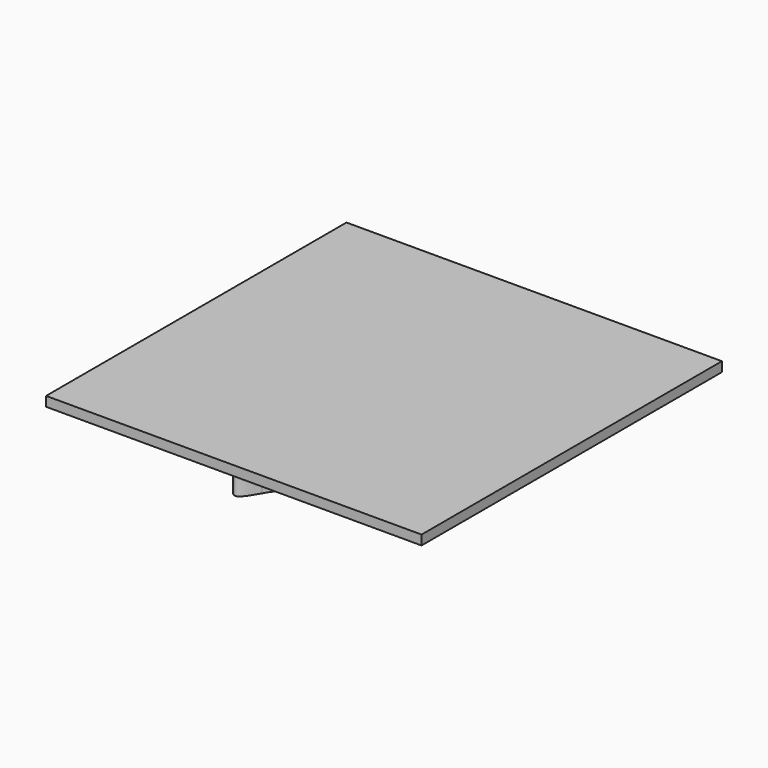
from build123d import *

# Parameters (mm, degrees)
F1_DEPTH = 25.4
F2_W     = 495.3
F2_H     = 495.3
F3_DEPTH = 12.7


# Not quite as in the source:
# - ends of sketch curves that miss each other by under 0.0002 mm in the source are joined


with BuildPart() as f1:
    # F0 (on Top) → F1 (new body)
    with BuildSketch(Plane.XY):
        with BuildLine():
            add(Edge.make_bspline(
                [(-4.6872398, -132.8896504), (2.565146, -134.5904598), (20.1811382, -134.4409808), (32.0904362, -132.5775352)],
                knots=[0, 0, 0, 0, 1, 1, 1, 1], degree=3))
            add(Edge.make_bspline(
                [(32.0904362, -132.5775352), (45.5382884, -130.47345), (63.2073666, -117.8832542), (63.2073666, -110.4049862)],
                knots=[0, 0, 0, 0, 1, 1, 1, 1], degree=3))
            add(Edge.make_bspline(
                [(63.2073666, -110.4049862), (63.2073666, -108.6564248), (65.2077436, -106.314367), (67.652646, -105.2003992)],
                knots=[0, 0, 0, 0, 1, 1, 1, 1], degree=3))
            add(Edge.make_bspline(
                [(67.652646, -105.2003992), (71.0041252, -103.6733512), (72.0979254, -101.8173224), (72.0979254, -97.657285)],
                knots=[0, 0, 0, 0, 1, 1, 1, 1], degree=3))
            add(Edge.make_bspline(
                [(72.0979254, -97.657285), (72.0979254, -93.98508), (74.1760264, -89.6034784), (78.3109432, -84.557362)],
                knots=[0, 0, 0, 0, 1, 1, 1, 1], degree=3))
            add(Edge.make_bspline(
                [(78.3109432, -84.557362), (81.7281068, -80.3871392), (85.0385396, -74.2513628), (85.667469, -70.922261)],
                knots=[0, 0, 0, 0, 1, 1, 1, 1], degree=3))
            add(Edge.make_bspline(
                [(85.667469, -70.922261), (86.2963476, -67.5931846), (88.1013732, -63.3937772), (89.6785608, -61.5902756)],
                knots=[0, 0, 0, 0, 1, 1, 1, 1], degree=3))
            add(Edge.make_bspline(
                [(89.6785608, -61.5902756), (96.3774298, -53.9301944), (96.9903826, -27.6993604), (90.744548, -15.9731456)],
                knots=[0, 0, 0, 0, 1, 1, 1, 1], degree=3))
            add(Edge.make_bspline(
                [(90.744548, -15.9731456), (89.441782, -13.5272526), (86.5961184, -7.5253342), (84.4208624, -2.6355294)],
                knots=[0, 0, 0, 0, 1, 1, 1, 1], degree=3))
            add(Edge.make_bspline(
                [(84.4208624, -2.6355294), (74.9756184, 18.5965592), (54.0221678, 33.8576666), (34.4270076, 33.7766914)],
                knots=[0, 0, 0, 0, 1, 1, 1, 1], degree=3))
            add(Edge.make_bspline(
                [(34.4270076, 33.7766914), (-6.2697868, 33.6084672), (-22.5027744, -13.94079), (3.7544248, -56.0687474)],
                knots=[0, 0, 0, 0, 1, 1, 1, 1], degree=3))
            add(Edge.make_bspline(
                [(3.7544248, -56.0687474), (14.4304766, -73.1977454), (11.871706, -79.905479), (-4.8053498, -78.5078948)],
                knots=[0, 0, 0, 0, 1, 1, 1, 1], degree=3))
            add(Edge.make_bspline(
                [(-4.8053498, -78.5078948), (-9.4479872, -78.1188684), (-8.5824822, -80.8853856), (-2.446274, -86.0486468)],
                knots=[0, 0, 0, 0, 1, 1, 1, 1], degree=3))
            add(Edge.make_bspline(
                [(-2.446274, -86.0486468), (8.1013808, -94.9239402), (29.9500798, -85.9176082), (26.9638526, -73.9254554)],
                knots=[0, 0, 0, 0, 1, 1, 1, 1], degree=3))
            add(Edge.make_bspline(
                [(26.9638526, -73.9254554), (23.0138224, -58.0628506), (23.357205, -56.3640224), (31.9564766, -49.2224314)],
                knots=[0, 0, 0, 0, 1, 1, 1, 1], degree=3))
            add(Edge.make_bspline(
                [(31.9564766, -49.2224314), (39.7350488, -42.7623986), (40.0891248, -42.060368), (40.027987, -33.2194408)],
                knots=[0, 0, 0, 0, 1, 1, 1, 1], degree=3))
            add(Edge.make_bspline(
                [(40.027987, -33.2194408), (39.9305272, -19.139281), (27.8596598, -6.8530216), (27.6723856, -20.6434436)],
                knots=[0, 0, 0, 0, 1, 1, 1, 1], degree=3))
            add(Edge.make_bspline(
                [(27.6723856, -20.6434436), (27.5848826, -27.0875252), (13.7894314, -30.181804), (8.956421, -24.8413778)],
                knots=[0, 0, 0, 0, 1, 1, 1, 1], degree=3))
            add(Edge.make_bspline(
                [(8.956421, -24.8413778), (-7.349109, -6.8239894), (33.8228686, 22.113367), (51.7718802, 5.2511198)],
                knots=[0, 0, 0, 0, 1, 1, 1, 1], degree=3))
            add(Edge.make_bspline(
                [(51.7718802, 5.2511198), (61.4420666, -3.8335204), (66.264282, -86.6088438), (57.9804022, -101.3206508)],
                knots=[0, 0, 0, 0, 1, 1, 1, 1], degree=3))
            add(Edge.make_bspline(
                [(57.9804022, -101.3206508), (56.6037476, -103.7655532), (54.984142, -108.1663826), (54.3812984, -111.1002604)],
                knots=[0, 0, 0, 0, 1, 1, 1, 1], degree=3))
            add(Edge.make_bspline(
                [(54.3812984, -111.1002604), (53.5451304, -115.1696706), (52.2480286, -116.500402), (48.9112052, -116.712111)],
                knots=[0, 0, 0, 0, 1, 1, 1, 1], degree=3))
            add(Edge.make_bspline(
                [(48.9112052, -116.712111), (46.505495, -116.8646634), (40.5364442, -117.438424), (35.6466394, -117.9869624)],
                knots=[0, 0, 0, 0, 1, 1, 1, 1], degree=3))
            add(Edge.make_bspline(
                [(35.6466394, -117.9869624), (15.5623006, -120.2399678), (-22.352635, -107.2693054), (-26.382853, -96.766761)],
                knots=[0, 0, 0, 0, 1, 1, 1, 1], degree=3))
            add(Edge.make_bspline(
                [(-26.382853, -96.766761), (-26.9341346, -95.3301878), (-29.3608252, -93.403674), (-31.7756032, -92.485591)],
                knots=[0, 0, 0, 0, 1, 1, 1, 1], degree=3))
            add(Edge.make_bspline(
                [(-31.7756032, -92.485591), (-34.1903304, -91.567508), (-38.0047246, -87.6215418), (-40.2519896, -83.7168252)],
                knots=[0, 0, 0, 0, 1, 1, 1, 1], degree=3))
            add(Edge.make_bspline(
                [(-40.2519896, -83.7168252), (-42.49928, -79.8120832), (-45.5450194, -76.2990346), (-47.0203022, -75.910059)],
                knots=[0, 0, 0, 0, 1, 1, 1, 1], degree=3))
            add(Edge.make_bspline(
                [(-47.0203022, -75.910059), (-48.495585, -75.5210834), (-51.2671568, -70.5764654), (-53.1793704, -64.922019)],
                knots=[0, 0, 0, 0, 1, 1, 1, 1], degree=3))
            add(Edge.make_bspline(
                [(-53.1793704, -64.922019), (-55.091584, -59.2675726), (-58.0647302, -52.850415), (-59.7864184, -50.661697)],
                knots=[0, 0, 0, 0, 1, 1, 1, 1], degree=3))
            add(Edge.make_bspline(
                [(-59.7864184, -50.661697), (-65.2226534, -43.7506364), (-71.3298294, -20.2546966), (-70.652005, -8.8589104)],
                knots=[0, 0, 0, 0, 1, 1, 1, 1], degree=3))
            add(Edge.make_bspline(
                [(-70.652005, -8.8589104), (-69.7677548, 6.0072016), (-65.1372586, 32.8197718), (-63.3513338, 33.415097)],
                knots=[0, 0, 0, 0, 1, 1, 1, 1], degree=3))
            add(Edge.make_bspline(
                [(-63.3513338, 33.415097), (-62.1608612, 33.8119466), (-61.260355, 37.5658888), (-61.260355, 42.131869)],
                knots=[0, 0, 0, 0, 1, 1, 1, 1], degree=3))
            add(Edge.make_bspline(
                [(-61.260355, 42.131869), (-61.260355, 48.5776778), (-60.5823274, 50.3289824), (-57.805701, 51.0550668)],
                knots=[0, 0, 0, 0, 1, 1, 1, 1], degree=3))
            add(Edge.make_bspline(
                [(-57.805701, 51.0550668), (-55.7726596, 51.5867142), (-53.874416, 54.1286192), (-53.1927562, 57.2321182)],
                knots=[0, 0, 0, 0, 1, 1, 1, 1], degree=3))
            add(Edge.make_bspline(
                [(-53.1927562, 57.2321182), (-52.555648, 60.1326458), (-50.9453642, 62.9237248), (-49.6142264, 63.4345188)],
                knots=[0, 0, 0, 0, 1, 1, 1, 1], degree=3))
            add(Edge.make_bspline(
                [(-49.6142264, 63.4345188), (-48.283114, 63.9453382), (-44.157773, 67.2333174), (-40.4468076, 70.7411336)],
                knots=[0, 0, 0, 0, 1, 1, 1, 1], degree=3))
            add(Edge.make_bspline(
                [(-40.4468076, 70.7411336), (-33.2821788, 77.5136372), (-5.460619, 91.604846), (-2.6650188, 89.8770872)],
                knots=[0, 0, 0, 0, 1, 1, 1, 1], degree=3))
            add(Edge.make_bspline(
                [(-2.6650188, 89.8770872), (-1.7519904, 89.3127754), (2.4407622, 85.224874), (6.6522092, 80.792828)],
                knots=[0, 0, 0, 0, 1, 1, 1, 1], degree=3))
            add(Edge.make_bspline(
                [(6.6522092, 80.792828), (28.443555, 57.8598792), (66.2333956, 48.0232974), (81.0458628, 61.4284014)],
                knots=[0, 0, 0, 0, 1, 1, 1, 1], degree=3))
            add(Edge.make_bspline(
                [(81.0458628, 61.4284014), (82.8469768, 63.0583702), (85.1039446, 63.9078224), (86.0613976, 63.316104)],
                knots=[0, 0, 0, 0, 1, 1, 1, 1], degree=3))
            add(Edge.make_bspline(
                [(86.0613976, 63.316104), (93.9387504, 58.4476606), (106.1099732, 90.8439382), (101.031421, 103.1620492)],
                knots=[0, 0, 0, 0, 1, 1, 1, 1], degree=3))
            add(Edge.make_bspline(
                [(101.031421, 103.1620492), (100.0234474, 105.6069262), (98.895281, 109.2076048), (98.5244156, 111.1635318)],
                knots=[0, 0, 0, 0, 1, 1, 1, 1], degree=3))
            add(Edge.make_bspline(
                [(98.5244156, 111.1635318), (98.076639, 113.5249444), (96.176211, 114.912267), (92.867988, 115.292759)],
                knots=[0, 0, 0, 0, 1, 1, 1, 1], degree=3))
            add(Edge.make_bspline(
                [(92.867988, 115.292759), (81.3739038, 116.6147274), (78.5806912, 104.2049224), (88.9899668, 98.063304)],
                knots=[0, 0, 0, 0, 1, 1, 1, 1], degree=3))
            add(Edge.make_bspline(
                [(88.9899668, 98.063304), (96.0866252, 93.8761648), (96.2397872, 93.3191682), (92.4067748, 85.6357444)],
                knots=[0, 0, 0, 0, 1, 1, 1, 1], degree=3))
            add(Edge.make_bspline(
                [(92.4067748, 85.6357444), (86.8952542, 74.5876334), (58.5066648, 79.412973), (44.0674506, 93.8521872)],
                knots=[0, 0, 0, 0, 1, 1, 1, 1], degree=3))
            add(Edge.make_bspline(
                [(44.0674506, 93.8521872), (40.2645372, 97.6550752), (35.8139492, 101.2804172), (34.1772494, 101.908483)],
                knots=[0, 0, 0, 0, 1, 1, 1, 1], degree=3))
            add(Edge.make_bspline(
                [(34.1772494, 101.908483), (32.5404988, 102.5365742), (31.2013854, 104.30764), (31.2013854, 105.8442384)],
                knots=[0, 0, 0, 0, 1, 1, 1, 1], degree=3))
            add(Edge.make_bspline(
                [(31.2013854, 105.8442384), (31.2013854, 115.9828262), (20.824317, 125.8578382), (15.6293566, 120.6628778)],
                knots=[0, 0, 0, 0, 1, 1, 1, 1], degree=3))
            add(Edge.make_bspline(
                [(15.6293566, 120.6628778), (12.5948186, 117.6283398), (8.415528, 121.7503026), (7.7441806, 128.4398498)],
                knots=[0, 0, 0, 0, 1, 1, 1, 1], degree=3))
            add(Edge.make_bspline(
                [(7.7441806, 128.4398498), (7.1968868, 133.8936108), (7.1968868, 133.8936108), (-1.152779, 127.503682)],
                knots=[0, 0, 0, 0, 1, 1, 1, 1], degree=3))
            add(Edge.make_bspline(
                [(-1.152779, 127.503682), (-5.745099, 123.989211), (-12.5463554, 119.4359816), (-16.2667188, 117.3853888)],
                knots=[0, 0, 0, 0, 1, 1, 1, 1], degree=3))
            add(Edge.make_bspline(
                [(-16.2667188, 117.3853888), (-29.5127426, 110.0844382), (-33.7114134, 107.5928252), (-34.588704, 106.5125886)],
                knots=[0, 0, 0, 0, 1, 1, 1, 1], degree=3))
            add(Edge.make_bspline(
                [(-34.588704, 106.5125886), (-35.0776794, 105.910507), (-38.8422388, 103.712264), (-42.9543972, 101.6276352)],
                knots=[0, 0, 0, 0, 1, 1, 1, 1], degree=3))
            add(Edge.make_bspline(
                [(-42.9543972, 101.6276352), (-63.9228846, 90.997786), (-92.5681918, 53.1264368), (-100.4275868, 25.643586)],
                knots=[0, 0, 0, 0, 1, 1, 1, 1], degree=3))
            add(Edge.make_bspline(
                [(-100.4275868, 25.643586), (-122.373009, -51.095529), (-84.2439006, -114.2322074), (-4.6872398, -132.8896504)],
                knots=[0, 0, 0, 0, 1, 1, 1, 1], degree=3))
        make_face()
    extrude(amount=F1_DEPTH)



with BuildPart() as f1b:
    # F0 (on Top) → F1, piece 2 (new body)
    with BuildSketch(Plane.XY):
        with BuildLine():
            add(Edge.make_bspline(
                [(-1.0196322, -238.6796598), (-2.4189944, -236.9682332), (-7.4832718, -229.6874756), (-12.2735848, -222.5002154)],
                knots=[0, 0, 0, 0, 1, 1, 1, 1], degree=3))
            add(Edge.make_bspline(
                [(22.2908622, -220.3237148), (10.6402378, -241.3161798), (4.8586898, -245.8688758), (-1.0196322, -238.6796598)],
                knots=[0, 0, 0, 0, 1, 1, 1, 1], degree=3))
            add(Edge.make_bspline(
                [(56.0949348, -194.4309802), (32.1195954, -204.467714), (30.3300384, -205.838425), (22.2908622, -220.3237148)],
                knots=[0, 0, 0, 0, 1, 1, 1, 1], degree=3))
            add(Edge.make_bspline(
                [(70.3197984, -187.5665032), (68.8528722, -188.680852), (62.4516658, -191.769873), (56.0949348, -194.4309802)],
                knots=[0, 0, 0, 0, 1, 1, 1, 1], degree=3))
            add(Edge.make_bspline(
                [(86.322789, -177.7426468), (78.9880818, -182.0314368), (71.78675, -186.4521798), (70.3197984, -187.5665032)],
                knots=[0, 0, 0, 0, 1, 1, 1, 1], degree=3))
            add(Edge.make_bspline(
                [(133.5823084, -146.0563754), (114.4429766, -160.1105256), (100.5704364, -169.4117008), (86.322789, -177.7426468)],
                knots=[0, 0, 0, 0, 1, 1, 1, 1], degree=3))
            add(Edge.make_bspline(
                [(153.2363712, -142.5615386), (145.4750202, -137.3234744), (145.4750202, -137.3234744), (133.5823084, -146.0563754)],
                knots=[0, 0, 0, 0, 1, 1, 1, 1], degree=3))
            add(Edge.make_bspline(
                [(198.6357216, -97.0345024), (167.2579586, -151.0684304), (166.6880588, -151.6399558), (153.2363712, -142.5615386)],
                knots=[0, 0, 0, 0, 1, 1, 1, 1], degree=3))
            add(Edge.make_bspline(
                [(206.1774388, -38.4766312), (224.3404708, -55.212742), (224.7447626, -52.0735814), (198.6357216, -97.0345024)],
                knots=[0, 0, 0, 0, 1, 1, 1, 1], degree=3))
            add(Edge.make_bspline(
                [(137.9170216, 86.2699824), (143.8160954, 42.9826928), (170.3009548, -5.4186836), (206.1774388, -38.4766312)],
                knots=[0, 0, 0, 0, 1, 1, 1, 1], degree=3))
            add(Edge.make_bspline(
                [(145.8894974, 104.067483), (135.0052926, 111.552609), (134.5960986, 110.6391234), (137.9170216, 86.2699824)],
                knots=[0, 0, 0, 0, 1, 1, 1, 1], degree=3))
            add(Edge.make_bspline(
                [(167.2346414, 100.9393968), (165.1424688, 95.842836), (155.8739834, 97.2011264), (145.8894974, 104.067483)],
                knots=[0, 0, 0, 0, 1, 1, 1, 1], degree=3))
            add(Edge.make_bspline(
                [(189.4531898, 170.2354482), (189.4531898, 166.9414238), (172.0588126, 112.691164), (167.2346414, 100.9393968)],
                knots=[0, 0, 0, 0, 1, 1, 1, 1], degree=3))
            add(Edge.make_bspline(
                [(119.630317, 241.8546344), (124.688727, 241.8546344), (189.4531898, 175.4239824), (189.4531898, 170.2354482)],
                knots=[0, 0, 0, 0, 1, 1, 1, 1], degree=3))
            add(Edge.make_bspline(
                [(82.1903868, 224.732977), (92.1461708, 231.5813504), (114.6107436, 241.8546344), (119.630317, 241.8546344)],
                knots=[0, 0, 0, 0, 1, 1, 1, 1], degree=3))
            add(Edge.make_bspline(
                [(71.2446632, 218.739212), (72.4724484, 218.739212), (77.397991, 221.4364126), (82.1903868, 224.732977)],
                knots=[0, 0, 0, 0, 1, 1, 1, 1], degree=3))
            add(Edge.make_bspline(
                [(56.7747912, 211.7525864), (63.5054356, 215.5952254), (70.0169034, 218.739212), (71.2446632, 218.739212)],
                knots=[0, 0, 0, 0, 1, 1, 1, 1], degree=3))
            add(Edge.make_bspline(
                [(-86.428707, 215.9315468), (6.7407028, 170.3246276), (-14.6936968, 170.950128), (56.7747912, 211.7525864)],
                knots=[0, 0, 0, 0, 1, 1, 1, 1], degree=3))
            add(Edge.make_bspline(
                [(-173.1847438, 194.603116), (-128.57607, 244.6274), (-139.5429772, 241.9312408), (-86.428707, 215.9315468)],
                knots=[0, 0, 0, 0, 1, 1, 1, 1], degree=3))
            add(Edge.make_bspline(
                [(-197.60946, 168.4192212), (-196.3205116, 169.2013126), (-185.3293982, 180.9840424), (-173.1847438, 194.603116)],
                knots=[0, 0, 0, 0, 1, 1, 1, 1], degree=3))
            add(Edge.make_bspline(
                [(-194.4519606, 142.8382462), (-200.3418904, 157.7141372), (-201.3807758, 166.1309606), (-197.60946, 168.4192212)],
                knots=[0, 0, 0, 0, 1, 1, 1, 1], degree=3))
            add(Edge.make_bspline(
                [(-178.8432288, 103.055674), (-182.637049, 112.9613946), (-184.2190626, 116.9934668), (-194.4519606, 142.8382462)],
                knots=[0, 0, 0, 0, 1, 1, 1, 1], degree=3))
            add(Edge.make_bspline(
                [(-150.6689392, 98.4466662), (-167.7549096, 83.567016), (-171.6214246, 84.1995522), (-178.8432288, 103.055674)],
                knots=[0, 0, 0, 0, 1, 1, 1, 1], degree=3))
            add(Edge.make_bspline(
                [(-143.7743886, 83.0520056), (-142.1342344, 102.718743), (-143.1525458, 104.9924748), (-150.6689392, 98.4466662)],
                knots=[0, 0, 0, 0, 1, 1, 1, 1], degree=3))
            add(Edge.make_bspline(
                [(-204.7925292, -46.1503014), (-169.9922432, -10.0557838), (-147.581874, 37.396801), (-143.7743886, 83.0520056)],
                knots=[0, 0, 0, 0, 1, 1, 1, 1], degree=3))
            add(Edge.make_bspline(
                [(-213.4781862, -79.0788614), (-222.31858, -66.0307544), (-221.7003186, -63.6868678), (-204.7925292, -46.1503014)],
                knots=[0, 0, 0, 0, 1, 1, 1, 1], degree=3))
            add(Edge.make_bspline(
                [(-185.0343772, -122.2134462), (-197.359778, -103.3877028), (-210.1594984, -83.9771498), (-213.4781862, -79.0788614)],
                knots=[0, 0, 0, 0, 1, 1, 1, 1], degree=3))
            add(Edge.make_bspline(
                [(-147.9286348, -150.2702608), (-160.5729072, -159.924877), (-160.1201776, -160.2671928), (-185.0343772, -122.2134462)],
                knots=[0, 0, 0, 0, 1, 1, 1, 1], degree=3))
            add(Edge.make_bspline(
                [(-134.9016606, -147.9874104), (-139.8456436, -144.0984672), (-139.8456436, -144.0984672), (-147.9286348, -150.2702608)],
                knots=[0, 0, 0, 0, 1, 1, 1, 1], degree=3))
            add(Edge.make_bspline(
                [(-26.4523982, -207.077056), (-61.5394248, -191.966215), (-118.3273478, -161.0247478), (-134.9016606, -147.9874104)],
                knots=[0, 0, 0, 0, 1, 1, 1, 1], degree=3))
            add(Edge.make_bspline(
                [(-12.2735848, -222.5002154), (-17.8885088, -214.0757212), (-22.9265734, -208.5955188), (-26.4523982, -207.077056)],
                knots=[0, 0, 0, 0, 1, 1, 1, 1], degree=3))
        make_face()
        with BuildLine():
            add(Edge.make_bspline(
                [(16.1130488, -218.0758402), (25.546177, -201.7135158), (29.5365932, -198.2191616), (46.0891382, -191.8259816)],
                knots=[0, 0, 0, 0, 1, 1, 1, 1], degree=3))
            add(Edge.make_bspline(
                [(-6.1952886, -219.6921946), (5.375148, -237.5706958), (4.8520604, -237.6085926), (16.1130488, -218.0758402)],
                knots=[0, 0, 0, 0, 1, 1, 1, 1], degree=3))
            add(Edge.make_bspline(
                [(-23.0309928, -201.6387128), (-17.3478952, -204.0591296), (-13.9645136, -207.6872402), (-6.1952886, -219.6921946)],
                knots=[0, 0, 0, 0, 1, 1, 1, 1], degree=3))
            add(Edge.make_bspline(
                [(-130.4374328, -143.361156), (-118.6673522, -153.5905996), (-55.964963, -187.6122486), (-23.0309928, -201.6387128)],
                knots=[0, 0, 0, 0, 1, 1, 1, 1], degree=3))
            add(Edge.make_bspline(
                [(-149.0571314, -143.0213802), (-140.9435586, -136.3729048), (-138.4253264, -136.4188534), (-130.4374328, -143.361156)],
                knots=[0, 0, 0, 0, 1, 1, 1, 1], degree=3))
            add(Edge.make_bspline(
                [(-174.0801446, -127.499745), (-158.0192674, -152.1953776), (-159.290512, -151.40686), (-149.0571314, -143.0213802)],
                knots=[0, 0, 0, 0, 1, 1, 1, 1], degree=3))
            add(Edge.make_bspline(
                [(-201.4165898, -85.7424498), (-194.1555934, -96.7553564), (-181.8541956, -115.5461494), (-174.0801446, -127.499745)],
                knots=[0, 0, 0, 0, 1, 1, 1, 1], degree=3))
            add(Edge.make_bspline(
                [(-203.2849122, -53.9206694), (-214.6183668, -65.718944), (-214.6183668, -65.718944), (-201.4165898, -85.7424498)],
                knots=[0, 0, 0, 0, 1, 1, 1, 1], degree=3))
            add(Edge.make_bspline(
                [(-188.4448098, -38.4315208), (-190.3734826, -40.4614888), (-197.0515236, -47.4316298), (-203.2849122, -53.9206694)],
                knots=[0, 0, 0, 0, 1, 1, 1, 1], degree=3))
            add(Edge.make_bspline(
                [(-153.7220954, 104.1752044), (-114.8346446, 138.4819176), (-147.3888594, 4.781296), (-188.4448098, -38.4315208)],
                knots=[0, 0, 0, 0, 1, 1, 1, 1], degree=3))
            add(Edge.make_bspline(
                [(-175.8733592, 112.9416334), (-167.7391108, 91.7735528), (-167.7671016, 91.7846272), (-153.7220954, 104.1752044)],
                knots=[0, 0, 0, 0, 1, 1, 1, 1], degree=3))
            add(Edge.make_bspline(
                [(-184.7594222, 135.1680304), (-182.5027084, 129.7892248), (-178.5039864, 119.7873652), (-175.8733592, 112.9416334)],
                knots=[0, 0, 0, 0, 1, 1, 1, 1], degree=3))
            add(Edge.make_bspline(
                [(-190.7703576, 165.665404), (-195.3905922, 160.8904326), (-195.248022, 160.167066), (-184.7594222, 135.1680304)],
                knots=[0, 0, 0, 0, 1, 1, 1, 1], degree=3))
            add(Edge.make_bspline(
                [(-160.8345272, 198.802879), (-175.0149662, 182.9380644), (-188.4860848, 168.026207), (-190.7703576, 165.665404)],
                knots=[0, 0, 0, 0, 1, 1, 1, 1], degree=3))
            add(Edge.make_bspline(
                [(-88.3770648, 209.835496), (-136.4728538, 233.3904908), (-128.886712, 234.5455812), (-160.8345272, 198.802879)],
                knots=[0, 0, 0, 0, 1, 1, 1, 1], degree=3))
            add(Edge.make_bspline(
                [(60.3309944, 206.4182562), (-14.7092162, 163.576635), (7.1000112, 163.0754676), (-88.3770648, 209.835496)],
                knots=[0, 0, 0, 0, 1, 1, 1, 1], degree=3))
            add(Edge.make_bspline(
                [(74.8008918, 213.4048818), (73.573132, 213.4048818), (67.0616642, 210.2608952), (60.3309944, 206.4182562)],
                knots=[0, 0, 0, 0, 1, 1, 1, 1], degree=3))
            add(Edge.make_bspline(
                [(85.717253, 219.3784538), (80.9410116, 216.0929892), (76.0286516, 213.4048818), (74.8008918, 213.4048818)],
                knots=[0, 0, 0, 0, 1, 1, 1, 1], degree=3))
            add(Edge.make_bspline(
                [(180.9865316, 173.2243678), (129.7037284, 233.2429422), (115.7206728, 240.017173), (85.717253, 219.3784538)],
                knots=[0, 0, 0, 0, 1, 1, 1, 1], degree=3))
            add(Edge.make_bspline(
                [(173.4463384, 137.8236512), (183.6627264, 168.3664654), (183.9569854, 169.7479206), (180.9865316, 173.2243678)],
                knots=[0, 0, 0, 0, 1, 1, 1, 1], degree=3))
            add(Edge.make_bspline(
                [(151.3781072, 108.2061082), (161.7070172, 101.2352052), (160.8009484, 100.0191548), (173.4463384, 137.8236512)],
                knots=[0, 0, 0, 0, 1, 1, 1, 1], degree=3))
            add(Edge.make_bspline(
                [(130.7823394, 103.3888458), (130.7715698, 119.614696), (133.5208912, 120.2577986), (151.3781072, 108.2061082)],
                knots=[0, 0, 0, 0, 1, 1, 1, 1], degree=3))
            add(Edge.make_bspline(
                [(200.9196134, -42.2138856), (158.5775086, -2.6710132), (130.81508, 54.9628822), (130.7823394, 103.3888458)],
                knots=[0, 0, 0, 0, 1, 1, 1, 1], degree=3))
            add(Edge.make_bspline(
                [(172.8439012, -127.677291), (219.508578, -50.5386848), (217.2372338, -57.4527426), (200.9196134, -42.2138856)],
                knots=[0, 0, 0, 0, 1, 1, 1, 1], degree=3))
            add(Edge.make_bspline(
                [(151.1132106, -133.1476382), (157.5652424, -143.5872668), (164.2349268, -141.9083014), (172.8439012, -127.677291)],
                knots=[0, 0, 0, 0, 1, 1, 1, 1], degree=3))
            add(Edge.make_bspline(
                [(130.0315916, -140.7400538), (141.9394418, -132.0478182), (148.887053, -129.5456642), (151.1132106, -133.1476382)],
                knots=[0, 0, 0, 0, 1, 1, 1, 1], degree=3))
            add(Edge.make_bspline(
                [(46.0891382, -191.8259816), (65.7315932, -184.2393826), (94.0487832, -167.006016), (130.0315916, -140.7400538)],
                knots=[0, 0, 0, 0, 1, 1, 1, 1], degree=3))
        make_face(mode=Mode.SUBTRACT)
        with BuildLine():
            add(Edge.make_bspline(
                [(-6.1952886, -219.6921946), (5.375148, -237.5706958), (4.8520604, -237.6085926), (16.1130488, -218.0758402)],
                knots=[0, 0, 0, 0, 1, 1, 1, 1], degree=3))
            add(Edge.make_bspline(
                [(16.1130488, -218.0758402), (25.546177, -201.7135158), (29.5365932, -198.2191616), (46.0891382, -191.8259816)],
                knots=[0, 0, 0, 0, 1, 1, 1, 1], degree=3))
            add(Edge.make_bspline(
                [(46.0891382, -191.8259816), (65.7315932, -184.2393826), (94.0487832, -167.006016), (130.0315916, -140.7400538)],
                knots=[0, 0, 0, 0, 1, 1, 1, 1], degree=3))
            add(Edge.make_bspline(
                [(130.0315916, -140.7400538), (141.9394418, -132.0478182), (148.887053, -129.5456642), (151.1132106, -133.1476382)],
                knots=[0, 0, 0, 0, 1, 1, 1, 1], degree=3))
            add(Edge.make_bspline(
                [(151.1132106, -133.1476382), (157.5652424, -143.5872668), (164.2349268, -141.9083014), (172.8439012, -127.677291)],
                knots=[0, 0, 0, 0, 1, 1, 1, 1], degree=3))
            add(Edge.make_bspline(
                [(172.8439012, -127.677291), (219.508578, -50.5386848), (217.2372338, -57.4527426), (200.9196134, -42.2138856)],
                knots=[0, 0, 0, 0, 1, 1, 1, 1], degree=3))
            add(Edge.make_bspline(
                [(200.9196134, -42.2138856), (158.5775086, -2.6710132), (130.81508, 54.9628822), (130.7823394, 103.3888458)],
                knots=[0, 0, 0, 0, 1, 1, 1, 1], degree=3))
            add(Edge.make_bspline(
                [(130.7823394, 103.3888458), (130.7715698, 119.614696), (133.5208912, 120.2577986), (151.3781072, 108.2061082)],
                knots=[0, 0, 0, 0, 1, 1, 1, 1], degree=3))
            add(Edge.make_bspline(
                [(151.3781072, 108.2061082), (161.7070172, 101.2352052), (160.8009484, 100.0191548), (173.4463384, 137.8236512)],
                knots=[0, 0, 0, 0, 1, 1, 1, 1], degree=3))
            add(Edge.make_bspline(
                [(173.4463384, 137.8236512), (183.6627264, 168.3664654), (183.9569854, 169.7479206), (180.9865316, 173.2243678)],
                knots=[0, 0, 0, 0, 1, 1, 1, 1], degree=3))
            add(Edge.make_bspline(
                [(180.9865316, 173.2243678), (129.7037284, 233.2429422), (115.7206728, 240.017173), (85.717253, 219.3784538)],
                knots=[0, 0, 0, 0, 1, 1, 1, 1], degree=3))
            add(Edge.make_bspline(
                [(85.717253, 219.3784538), (80.9410116, 216.0929892), (76.0286516, 213.4048818), (74.8008918, 213.4048818)],
                knots=[0, 0, 0, 0, 1, 1, 1, 1], degree=3))
            add(Edge.make_bspline(
                [(74.8008918, 213.4048818), (73.573132, 213.4048818), (67.0616642, 210.2608952), (60.3309944, 206.4182562)],
                knots=[0, 0, 0, 0, 1, 1, 1, 1], degree=3))
            add(Edge.make_bspline(
                [(60.3309944, 206.4182562), (-14.7092162, 163.576635), (7.1000112, 163.0754676), (-88.3770648, 209.835496)],
                knots=[0, 0, 0, 0, 1, 1, 1, 1], degree=3))
            add(Edge.make_bspline(
                [(-88.3770648, 209.835496), (-136.4728538, 233.3904908), (-128.886712, 234.5455812), (-160.8345272, 198.802879)],
                knots=[0, 0, 0, 0, 1, 1, 1, 1], degree=3))
            add(Edge.make_bspline(
                [(-160.8345272, 198.802879), (-175.0149662, 182.9380644), (-188.4860848, 168.026207), (-190.7703576, 165.665404)],
                knots=[0, 0, 0, 0, 1, 1, 1, 1], degree=3))
            add(Edge.make_bspline(
                [(-190.7703576, 165.665404), (-195.3905922, 160.8904326), (-195.248022, 160.167066), (-184.7594222, 135.1680304)],
                knots=[0, 0, 0, 0, 1, 1, 1, 1], degree=3))
            add(Edge.make_bspline(
                [(-184.7594222, 135.1680304), (-182.5027084, 129.7892248), (-178.5039864, 119.7873652), (-175.8733592, 112.9416334)],
                knots=[0, 0, 0, 0, 1, 1, 1, 1], degree=3))
            add(Edge.make_bspline(
                [(-175.8733592, 112.9416334), (-167.7391108, 91.7735528), (-167.7671016, 91.7846272), (-153.7220954, 104.1752044)],
                knots=[0, 0, 0, 0, 1, 1, 1, 1], degree=3))
            add(Edge.make_bspline(
                [(-153.7220954, 104.1752044), (-114.8346446, 138.4819176), (-147.3888594, 4.781296), (-188.4448098, -38.4315208)],
                knots=[0, 0, 0, 0, 1, 1, 1, 1], degree=3))
            add(Edge.make_bspline(
                [(-188.4448098, -38.4315208), (-190.3734826, -40.4614888), (-197.0515236, -47.4316298), (-203.2849122, -53.9206694)],
                knots=[0, 0, 0, 0, 1, 1, 1, 1], degree=3))
            add(Edge.make_bspline(
                [(-203.2849122, -53.9206694), (-214.6183668, -65.718944), (-214.6183668, -65.718944), (-201.4165898, -85.7424498)],
                knots=[0, 0, 0, 0, 1, 1, 1, 1], degree=3))
            add(Edge.make_bspline(
                [(-201.4165898, -85.7424498), (-194.1555934, -96.7553564), (-181.8541956, -115.5461494), (-174.0801446, -127.499745)],
                knots=[0, 0, 0, 0, 1, 1, 1, 1], degree=3))
            add(Edge.make_bspline(
                [(-174.0801446, -127.499745), (-158.0192674, -152.1953776), (-159.290512, -151.40686), (-149.0571314, -143.0213802)],
                knots=[0, 0, 0, 0, 1, 1, 1, 1], degree=3))
            add(Edge.make_bspline(
                [(-149.0571314, -143.0213802), (-140.9435586, -136.3729048), (-138.4253264, -136.4188534), (-130.4374328, -143.361156)],
                knots=[0, 0, 0, 0, 1, 1, 1, 1], degree=3))
            add(Edge.make_bspline(
                [(-130.4374328, -143.361156), (-118.6673522, -153.5905996), (-55.964963, -187.6122486), (-23.0309928, -201.6387128)],
                knots=[0, 0, 0, 0, 1, 1, 1, 1], degree=3))
            add(Edge.make_bspline(
                [(-23.0309928, -201.6387128), (-17.3478952, -204.0591296), (-13.9645136, -207.6872402), (-6.1952886, -219.6921946)],
                knots=[0, 0, 0, 0, 1, 1, 1, 1], degree=3))
        make_face()
        with BuildLine():
            add(Edge.make_bspline(
                [(15.6967428, -200.9136952), (4.6928024, -215.8597664), (4.7931832, -215.8187454), (-2.274951, -208.2559462)],
                knots=[0, 0, 0, 0, 1, 1, 1, 1], degree=3))
            add(Edge.make_bspline(
                [(-2.274951, -208.2559462), (-4.8891444, -205.458822), (-8.391017, -201.1568748), (-10.0569776, -198.6960466)],
                knots=[0, 0, 0, 0, 1, 1, 1, 1], degree=3))
            add(Edge.make_bspline(
                [(-10.0569776, -198.6960466), (-12.0608598, -195.7360068), (-18.6801506, -191.9944344), (-29.6161714, -187.6401886)],
                knots=[0, 0, 0, 0, 1, 1, 1, 1], degree=3))
            add(Edge.make_bspline(
                [(-29.6161714, -187.6401886), (-47.623984, -180.4702258), (-72.4833196, -167.6049988), (-98.7214688, -151.8767346)],
                knots=[0, 0, 0, 0, 1, 1, 1, 1], degree=3))
            add(Edge.make_bspline(
                [(-98.7214688, -151.8767346), (-107.9456566, -146.3473324), (-117.778149, -140.5116824), (-120.5714378, -138.908536)],
                knots=[0, 0, 0, 0, 1, 1, 1, 1], degree=3))
            add(Edge.make_bspline(
                [(-120.5714378, -138.908536), (-123.3647266, -137.3054404), (-129.2765766, -133.1403484), (-133.7088512, -129.6528268)],
                knots=[0, 0, 0, 0, 1, 1, 1, 1], degree=3))
            add(Edge.make_bspline(
                [(-133.7088512, -129.6528268), (-141.76756, -123.3118438), (-141.76756, -123.3118438), (-145.8858906, -127.4301998)],
                knots=[0, 0, 0, 0, 1, 1, 1, 1], degree=3))
            add(Edge.make_bspline(
                [(-145.8858906, -127.4301998), (-156.3296086, -137.8738924), (-158.6444884, -136.0450924), (-184.1034926, -97.237296)],
                knots=[0, 0, 0, 0, 1, 1, 1, 1], degree=3))
            add(Edge.make_bspline(
                [(-184.1034926, -97.237296), (-206.5406588, -63.0357896), (-206.2161738, -66.2009598), (-189.1446814, -48.0647248)],
                knots=[0, 0, 0, 0, 1, 1, 1, 1], degree=3))
            add(Edge.make_bspline(
                [(-189.1446814, -48.0647248), (-146.8589138, -3.141599), (-127.6927596, 46.3485992), (-124.5949756, 118.613428)],
                knots=[0, 0, 0, 0, 1, 1, 1, 1], degree=3))
            add(Edge.make_bspline(
                [(-124.5949756, 118.613428), (-123.742069, 138.5100862), (-123.742069, 138.5100862), (-134.7313282, 129.6439368)],
                knots=[0, 0, 0, 0, 1, 1, 1, 1], degree=3))
            add(Edge.make_bspline(
                [(-134.7313282, 129.6439368), (-158.2743596, 110.6494104), (-164.964745, 109.0582782), (-169.7329092, 121.3197218)],
                knots=[0, 0, 0, 0, 1, 1, 1, 1], degree=3))
            add(Edge.make_bspline(
                [(-169.7329092, 121.3197218), (-174.9382328, 134.7052932), (-180.9066486, 148.8048332), (-183.2379622, 153.223468)],
                knots=[0, 0, 0, 0, 1, 1, 1, 1], degree=3))
            add(Edge.make_bspline(
                [(-183.2379622, 153.223468), (-186.638692, 159.6690228), (-187.0431362, 158.7765684), (-174.6148908, 172.2508874)],
                knots=[0, 0, 0, 0, 1, 1, 1, 1], degree=3))
            add(Edge.make_bspline(
                [(-174.6148908, 172.2508874), (-168.5026348, 178.877595), (-157.1004986, 191.6386058), (-149.276816, 200.608692)],
                knots=[0, 0, 0, 0, 1, 1, 1, 1], degree=3))
            add(Edge.make_bspline(
                [(-149.276816, 200.608692), (-130.9323518, 221.641162), (-132.6471566, 221.4193692), (-102.9322808, 206.6027364)],
                knots=[0, 0, 0, 0, 1, 1, 1, 1], degree=3))
            add(Edge.make_bspline(
                [(-102.9322808, 206.6027364), (-81.2557938, 195.794249), (-61.185425, 186.0662014), (-17.0812206, 164.9909578)],
                knots=[0, 0, 0, 0, 1, 1, 1, 1], degree=3))
            add(Edge.make_bspline(
                [(-17.0812206, 164.9909578), (-5.7971182, 159.5988426), (-5.7971182, 159.5988426), (0.699897, 163.1695492)],
                knots=[0, 0, 0, 0, 1, 1, 1, 1], degree=3))
            add(Edge.make_bspline(
                [(0.699897, 163.1695492), (4.2732198, 165.1334518), (16.7986964, 172.0960744), (28.5342076, 178.6420354)],
                knots=[0, 0, 0, 0, 1, 1, 1, 1], degree=3))
            add(Edge.make_bspline(
                [(28.5342076, 178.6420354), (53.3757886, 192.4984466), (50.7144274, 191.0329682), (86.783926, 210.7173078)],
                knots=[0, 0, 0, 0, 1, 1, 1, 1], degree=3))
            add(Edge.make_bspline(
                [(86.783926, 210.7173078), (117.7499042, 227.6164866), (115.6905484, 227.4361466), (127.625856, 214.2939326)],
                knots=[0, 0, 0, 0, 1, 1, 1, 1], degree=3))
            add(Edge.make_bspline(
                [(127.625856, 214.2939326), (132.0666142, 209.4041278), (143.8000934, 197.1665602), (153.700226, 187.0993464)],
                knots=[0, 0, 0, 0, 1, 1, 1, 1], degree=3))
            add(Edge.make_bspline(
                [(153.700226, 187.0993464), (174.0919302, 166.363523), (173.2287366, 169.8240698), (164.3836184, 144.2695362)],
                knots=[0, 0, 0, 0, 1, 1, 1, 1], degree=3))
            add(Edge.make_bspline(
                [(164.3836184, 144.2695362), (161.5465654, 136.0729054), (159.2253102, 127.8462518), (159.2253102, 125.9880894)],
                knots=[0, 0, 0, 0, 1, 1, 1, 1], degree=3))
            add(Edge.make_bspline(
                [(159.2253102, 125.9880894), (159.2253102, 117.5626808), (144.8010312, 122.1656688), (125.4412274, 136.7690686)],
                knots=[0, 0, 0, 0, 1, 1, 1, 1], degree=3))
            add(Edge.make_bspline(
                [(125.4412274, 136.7690686), (114.025553, 145.3801004), (111.3929446, 139.6929642), (114.8229098, 113.8307096)],
                knots=[0, 0, 0, 0, 1, 1, 1, 1], degree=3))
            add(Edge.make_bspline(
                [(114.8229098, 113.8307096), (115.795679, 106.4960024), (116.9261314, 97.2942682), (117.335046, 93.3824142)],
                knots=[0, 0, 0, 0, 1, 1, 1, 1], degree=3))
            add(Edge.make_bspline(
                [(117.335046, 93.3824142), (122.2379826, 46.4773518), (149.8361748, -4.9135538), (191.4757664, -44.6759076)],
                knots=[0, 0, 0, 0, 1, 1, 1, 1], degree=3))
            add(Edge.make_bspline(
                [(191.4757664, -44.6759076), (203.9539736, -56.5915302), (204.194156, -55.5762668), (178.92649, -97.7251792)],
                knots=[0, 0, 0, 0, 1, 1, 1, 1], degree=3))
            add(Edge.make_bspline(
                [(178.92649, -97.7251792), (171.0247024, -110.9060266), (164.5596404, -122.3081628), (164.5596404, -123.0632286)],
                knots=[0, 0, 0, 0, 1, 1, 1, 1], degree=3))
            add(Edge.make_bspline(
                [(164.5596404, -123.0632286), (164.5596404, -126.001399), (156.6122852, -124.2213416), (151.1586258, -120.0616344)],
                knots=[0, 0, 0, 0, 1, 1, 1, 1], degree=3))
            add(Edge.make_bspline(
                [(151.1586258, -120.0616344), (145.4234074, -115.6871702), (145.4234074, -115.6871702), (142.1631904, -119.289703)],
                knots=[0, 0, 0, 0, 1, 1, 1, 1], degree=3))
            add(Edge.make_bspline(
                [(142.1631904, -119.289703), (140.370052, -121.2710808), (133.6736468, -126.4759218), (127.2822702, -130.8560248)],
                knots=[0, 0, 0, 0, 1, 1, 1, 1], degree=3))
            add(Edge.make_bspline(
                [(127.2822702, -130.8560248), (120.890919, -135.2361024), (108.0601852, -144.0438826), (98.7695764, -150.4288076)],
                knots=[0, 0, 0, 0, 1, 1, 1, 1], degree=3))
            add(Edge.make_bspline(
                [(98.7695764, -150.4288076), (89.4789422, -156.813758), (77.4767056, -164.4026684), (72.0979254, -167.293036)],
                knots=[0, 0, 0, 0, 1, 1, 1, 1], degree=3))
            add(Edge.make_bspline(
                [(72.0979254, -167.293036), (66.7191198, -170.183429), (58.513853, -174.9043238), (53.8639512, -177.7839472)],
                knots=[0, 0, 0, 0, 1, 1, 1, 1], degree=3))
            add(Edge.make_bspline(
                [(53.8639512, -177.7839472), (49.2140748, -180.6635706), (40.0465544, -185.2497184), (33.4917542, -187.975367)],
                knots=[0, 0, 0, 0, 1, 1, 1, 1], degree=3))
            add(Edge.make_bspline(
                [(33.4917542, -187.975367), (24.1788442, -191.8479018), (20.289266, -194.6759124), (15.6967428, -200.9136952)],
                knots=[0, 0, 0, 0, 1, 1, 1, 1], degree=3))
        make_face(mode=Mode.SUBTRACT)
        with BuildLine():
            add(Edge.make_bspline(
                [(-2.274951, -208.2559462), (-4.8891444, -205.458822), (-8.391017, -201.1568748), (-10.0569776, -198.6960466)],
                knots=[0, 0, 0, 0, 1, 1, 1, 1], degree=3))
            add(Edge.make_bspline(
                [(15.6967428, -200.9136952), (4.6928024, -215.8597664), (4.7931832, -215.8187454), (-2.274951, -208.2559462)],
                knots=[0, 0, 0, 0, 1, 1, 1, 1], degree=3))
            add(Edge.make_bspline(
                [(33.4917542, -187.975367), (24.1788442, -191.8479018), (20.289266, -194.6759124), (15.6967428, -200.9136952)],
                knots=[0, 0, 0, 0, 1, 1, 1, 1], degree=3))
            add(Edge.make_bspline(
                [(53.8639512, -177.7839472), (49.2140748, -180.6635706), (40.0465544, -185.2497184), (33.4917542, -187.975367)],
                knots=[0, 0, 0, 0, 1, 1, 1, 1], degree=3))
            add(Edge.make_bspline(
                [(72.0979254, -167.293036), (66.7191198, -170.183429), (58.513853, -174.9043238), (53.8639512, -177.7839472)],
                knots=[0, 0, 0, 0, 1, 1, 1, 1], degree=3))
            add(Edge.make_bspline(
                [(98.7695764, -150.4288076), (89.4789422, -156.813758), (77.4767056, -164.4026684), (72.0979254, -167.293036)],
                knots=[0, 0, 0, 0, 1, 1, 1, 1], degree=3))
            add(Edge.make_bspline(
                [(127.2822702, -130.8560248), (120.890919, -135.2361024), (108.0601852, -144.0438826), (98.7695764, -150.4288076)],
                knots=[0, 0, 0, 0, 1, 1, 1, 1], degree=3))
            add(Edge.make_bspline(
                [(142.1631904, -119.289703), (140.370052, -121.2710808), (133.6736468, -126.4759218), (127.2822702, -130.8560248)],
                knots=[0, 0, 0, 0, 1, 1, 1, 1], degree=3))
            add(Edge.make_bspline(
                [(151.1586258, -120.0616344), (145.4234074, -115.6871702), (145.4234074, -115.6871702), (142.1631904, -119.289703)],
                knots=[0, 0, 0, 0, 1, 1, 1, 1], degree=3))
            add(Edge.make_bspline(
                [(164.5596404, -123.0632286), (164.5596404, -126.001399), (156.6122852, -124.2213416), (151.1586258, -120.0616344)],
                knots=[0, 0, 0, 0, 1, 1, 1, 1], degree=3))
            add(Edge.make_bspline(
                [(178.92649, -97.7251792), (171.0247024, -110.9060266), (164.5596404, -122.3081628), (164.5596404, -123.0632286)],
                knots=[0, 0, 0, 0, 1, 1, 1, 1], degree=3))
            add(Edge.make_bspline(
                [(191.4757664, -44.6759076), (203.9539736, -56.5915302), (204.194156, -55.5762668), (178.92649, -97.7251792)],
                knots=[0, 0, 0, 0, 1, 1, 1, 1], degree=3))
            add(Edge.make_bspline(
                [(117.335046, 93.3824142), (122.2379826, 46.4773518), (149.8361748, -4.9135538), (191.4757664, -44.6759076)],
                knots=[0, 0, 0, 0, 1, 1, 1, 1], degree=3))
            add(Edge.make_bspline(
                [(114.8229098, 113.8307096), (115.795679, 106.4960024), (116.9261314, 97.2942682), (117.335046, 93.3824142)],
                knots=[0, 0, 0, 0, 1, 1, 1, 1], degree=3))
            add(Edge.make_bspline(
                [(125.4412274, 136.7690686), (114.025553, 145.3801004), (111.3929446, 139.6929642), (114.8229098, 113.8307096)],
                knots=[0, 0, 0, 0, 1, 1, 1, 1], degree=3))
            add(Edge.make_bspline(
                [(159.2253102, 125.9880894), (159.2253102, 117.5626808), (144.8010312, 122.1656688), (125.4412274, 136.7690686)],
                knots=[0, 0, 0, 0, 1, 1, 1, 1], degree=3))
            add(Edge.make_bspline(
                [(164.3836184, 144.2695362), (161.5465654, 136.0729054), (159.2253102, 127.8462518), (159.2253102, 125.9880894)],
                knots=[0, 0, 0, 0, 1, 1, 1, 1], degree=3))
            add(Edge.make_bspline(
                [(153.700226, 187.0993464), (174.0919302, 166.363523), (173.2287366, 169.8240698), (164.3836184, 144.2695362)],
                knots=[0, 0, 0, 0, 1, 1, 1, 1], degree=3))
            add(Edge.make_bspline(
                [(127.625856, 214.2939326), (132.0666142, 209.4041278), (143.8000934, 197.1665602), (153.700226, 187.0993464)],
                knots=[0, 0, 0, 0, 1, 1, 1, 1], degree=3))
            add(Edge.make_bspline(
                [(86.783926, 210.7173078), (117.7499042, 227.6164866), (115.6905484, 227.4361466), (127.625856, 214.2939326)],
                knots=[0, 0, 0, 0, 1, 1, 1, 1], degree=3))
            add(Edge.make_bspline(
                [(28.5342076, 178.6420354), (53.3757886, 192.4984466), (50.7144274, 191.0329682), (86.783926, 210.7173078)],
                knots=[0, 0, 0, 0, 1, 1, 1, 1], degree=3))
            add(Edge.make_bspline(
                [(0.699897, 163.1695492), (4.2732198, 165.1334518), (16.7986964, 172.0960744), (28.5342076, 178.6420354)],
                knots=[0, 0, 0, 0, 1, 1, 1, 1], degree=3))
            add(Edge.make_bspline(
                [(-17.0812206, 164.9909578), (-5.7971182, 159.5988426), (-5.7971182, 159.5988426), (0.699897, 163.1695492)],
                knots=[0, 0, 0, 0, 1, 1, 1, 1], degree=3))
            add(Edge.make_bspline(
                [(-102.9322808, 206.6027364), (-81.2557938, 195.794249), (-61.185425, 186.0662014), (-17.0812206, 164.9909578)],
                knots=[0, 0, 0, 0, 1, 1, 1, 1], degree=3))
            add(Edge.make_bspline(
                [(-149.276816, 200.608692), (-130.9323518, 221.641162), (-132.6471566, 221.4193692), (-102.9322808, 206.6027364)],
                knots=[0, 0, 0, 0, 1, 1, 1, 1], degree=3))
            add(Edge.make_bspline(
                [(-174.6148908, 172.2508874), (-168.5026348, 178.877595), (-157.1004986, 191.6386058), (-149.276816, 200.608692)],
                knots=[0, 0, 0, 0, 1, 1, 1, 1], degree=3))
            add(Edge.make_bspline(
                [(-183.2379622, 153.223468), (-186.638692, 159.6690228), (-187.0431362, 158.7765684), (-174.6148908, 172.2508874)],
                knots=[0, 0, 0, 0, 1, 1, 1, 1], degree=3))
            add(Edge.make_bspline(
                [(-169.7329092, 121.3197218), (-174.9382328, 134.7052932), (-180.9066486, 148.8048332), (-183.2379622, 153.223468)],
                knots=[0, 0, 0, 0, 1, 1, 1, 1], degree=3))
            add(Edge.make_bspline(
                [(-134.7313282, 129.6439368), (-158.2743596, 110.6494104), (-164.964745, 109.0582782), (-169.7329092, 121.3197218)],
                knots=[0, 0, 0, 0, 1, 1, 1, 1], degree=3))
            add(Edge.make_bspline(
                [(-124.5949756, 118.613428), (-123.742069, 138.5100862), (-123.742069, 138.5100862), (-134.7313282, 129.6439368)],
                knots=[0, 0, 0, 0, 1, 1, 1, 1], degree=3))
            add(Edge.make_bspline(
                [(-189.1446814, -48.0647248), (-146.8589138, -3.141599), (-127.6927596, 46.3485992), (-124.5949756, 118.613428)],
                knots=[0, 0, 0, 0, 1, 1, 1, 1], degree=3))
            add(Edge.make_bspline(
                [(-184.1034926, -97.237296), (-206.5406588, -63.0357896), (-206.2161738, -66.2009598), (-189.1446814, -48.0647248)],
                knots=[0, 0, 0, 0, 1, 1, 1, 1], degree=3))
            add(Edge.make_bspline(
                [(-145.8858906, -127.4301998), (-156.3296086, -137.8738924), (-158.6444884, -136.0450924), (-184.1034926, -97.237296)],
                knots=[0, 0, 0, 0, 1, 1, 1, 1], degree=3))
            add(Edge.make_bspline(
                [(-133.7088512, -129.6528268), (-141.76756, -123.3118438), (-141.76756, -123.3118438), (-145.8858906, -127.4301998)],
                knots=[0, 0, 0, 0, 1, 1, 1, 1], degree=3))
            add(Edge.make_bspline(
                [(-120.5714378, -138.908536), (-123.3647266, -137.3054404), (-129.2765766, -133.1403484), (-133.7088512, -129.6528268)],
                knots=[0, 0, 0, 0, 1, 1, 1, 1], degree=3))
            add(Edge.make_bspline(
                [(-98.7214688, -151.8767346), (-107.9456566, -146.3473324), (-117.778149, -140.5116824), (-120.5714378, -138.908536)],
                knots=[0, 0, 0, 0, 1, 1, 1, 1], degree=3))
            add(Edge.make_bspline(
                [(-29.6161714, -187.6401886), (-47.623984, -180.4702258), (-72.4833196, -167.6049988), (-98.7214688, -151.8767346)],
                knots=[0, 0, 0, 0, 1, 1, 1, 1], degree=3))
            add(Edge.make_bspline(
                [(-10.0569776, -198.6960466), (-12.0608598, -195.7360068), (-18.6801506, -191.9944344), (-29.6161714, -187.6401886)],
                knots=[0, 0, 0, 0, 1, 1, 1, 1], degree=3))
        make_face()
        with BuildLine():
            add(Edge.make_bspline(
                [(13.8928348, -192.6687028), (16.7337486, -189.4088668), (23.5458508, -185.130059), (30.0228762, -182.5371254)],
                knots=[0, 0, 0, 0, 1, 1, 1, 1], degree=3))
            add(Edge.make_bspline(
                [(6.129528, -202.656821), (7.694549, -200.2670112), (11.1880142, -195.7723288), (13.8928348, -192.6687028)],
                knots=[0, 0, 0, 0, 1, 1, 1, 1], degree=3))
            add(Edge.make_bspline(
                [(-1.4213586, -199.5480642), (3.284093, -207.0019482), (3.284093, -207.0019482), (6.129528, -202.656821)],
                knots=[0, 0, 0, 0, 1, 1, 1, 1], degree=3))
            add(Edge.make_bspline(
                [(-28.365323, -181.3310318), (-10.0870766, -188.515625), (-7.1190612, -190.5223266), (-1.4213586, -199.5480642)],
                knots=[0, 0, 0, 0, 1, 1, 1, 1], degree=3))
            add(Edge.make_bspline(
                [(-95.1652402, -146.542379), (-69.5838334, -161.8769686), (-44.1189618, -175.1387912), (-28.365323, -181.3310318)],
                knots=[0, 0, 0, 0, 1, 1, 1, 1], degree=3))
            add(Edge.make_bspline(
                [(-117.0032204, -133.5741804), (-114.2165102, -135.1773268), (-104.389428, -141.0129768), (-95.1652402, -146.542379)],
                knots=[0, 0, 0, 0, 1, 1, 1, 1], degree=3))
            add(Edge.make_bspline(
                [(-130.593592, -123.9915224), (-125.9055648, -127.658876), (-119.7899052, -131.9710848), (-117.0032204, -133.5741804)],
                knots=[0, 0, 0, 0, 1, 1, 1, 1], degree=3))
            add(Edge.make_bspline(
                [(-149.4325434, -121.7688954), (-143.8705022, -115.767358), (-140.615797, -116.1513298), (-130.593592, -123.9915224)],
                knots=[0, 0, 0, 0, 1, 1, 1, 1], degree=3))
            add(Edge.make_bspline(
                [(-155.3948378, -126.2141748), (-154.381454, -126.2141748), (-151.6984012, -124.2137978), (-149.4325434, -121.7688954)],
                knots=[0, 0, 0, 0, 1, 1, 1, 1], degree=3))
            add(Edge.make_bspline(
                [(-196.1076088, -67.0703256), (-193.516758, -72.923146), (-156.8328842, -126.2141748), (-155.3948378, -126.2141748)],
                knots=[0, 0, 0, 0, 1, 1, 1, 1], degree=3))
            add(Edge.make_bspline(
                [(-184.2409574, -52.3659608), (-191.0975858, -59.7079578), (-196.4375802, -66.3249372), (-196.1076088, -67.0703256)],
                knots=[0, 0, 0, 0, 1, 1, 1, 1], degree=3))
            add(Edge.make_bspline(
                [(-118.8970952, 120.4986414), (-121.9419964, 43.5598316), (-140.4961376, -5.5244238), (-184.2409574, -52.3659608)],
                knots=[0, 0, 0, 0, 1, 1, 1, 1], degree=3))
            add(Edge.make_bspline(
                [(-133.6647314, 138.7516402), (-118.9604428, 151.694896), (-117.723031, 150.165435), (-118.8970952, 120.4986414)],
                knots=[0, 0, 0, 0, 1, 1, 1, 1], degree=3))
            add(Edge.make_bspline(
                [(-161.364676, 119.1650652), (-159.527367, 119.1650652), (-141.1684756, 132.1465988), (-133.6647314, 138.7516402)],
                knots=[0, 0, 0, 0, 1, 1, 1, 1], degree=3))
            add(Edge.make_bspline(
                [(-164.4267476, 124.9439208), (-163.191698, 121.7655426), (-161.8137734, 119.1650652), (-161.364676, 119.1650652)],
                knots=[0, 0, 0, 0, 1, 1, 1, 1], degree=3))
            add(Edge.make_bspline(
                [(-177.1254014, 155.3401262), (-175.4542084, 152.172797), (-169.058209, 136.8629724), (-164.4267476, 124.9439208)],
                knots=[0, 0, 0, 0, 1, 1, 1, 1], degree=3))
            add(Edge.make_bspline(
                [(-168.5117026, 169.6626528), (-177.0015764, 160.599755), (-178.5457694, 158.0321452), (-177.1254014, 155.3401262)],
                knots=[0, 0, 0, 0, 1, 1, 1, 1], degree=3))
            add(Edge.make_bspline(
                [(-144.8315366, 196.038978), (-152.1662438, 187.6053652), (-162.8223312, 175.7360214), (-168.5117026, 169.6626528)],
                knots=[0, 0, 0, 0, 1, 1, 1, 1], degree=3))
            add(Edge.make_bspline(
                [(-104.7226506, 200.287255), (-132.6838088, 214.0643674), (-128.796796, 214.476076), (-144.8315366, 196.038978)],
                knots=[0, 0, 0, 0, 1, 1, 1, 1], degree=3))
            add(Edge.make_bspline(
                [(-21.112353, 159.8880216), (-54.8770048, 176.008665), (-84.3919826, 190.269876), (-104.7226506, 200.287255)],
                knots=[0, 0, 0, 0, 1, 1, 1, 1], degree=3))
            add(Edge.make_bspline(
                [(-5.8097674, 154.727275), (-8.2811366, 154.727275), (-15.1673052, 157.049597), (-21.112353, 159.8880216)],
                knots=[0, 0, 0, 0, 1, 1, 1, 1], degree=3))
            add(Edge.make_bspline(
                [(54.3168078, 185.8848708), (47.9779584, 180.484399), (-1.7270222, 154.727275), (-5.8097674, 154.727275)],
                knots=[0, 0, 0, 0, 1, 1, 1, 1], degree=3))
            add(Edge.make_bspline(
                [(63.2073666, 190.7355596), (59.784488, 189.3174522), (55.7837594, 187.1346524), (54.3168078, 185.8848708)],
                knots=[0, 0, 0, 0, 1, 1, 1, 1], degree=3))
            add(Edge.make_bspline(
                [(92.1017716, 206.0315666), (79.6327084, 199.0368384), (66.6302198, 192.1536416), (63.2073666, 190.7355596)],
                knots=[0, 0, 0, 0, 1, 1, 1, 1], degree=3))
            add(Edge.make_bspline(
                [(121.440575, 211.2289654), (114.7727956, 218.7492196), (114.7727956, 218.7492196), (92.1017716, 206.0315666)],
                knots=[0, 0, 0, 0, 1, 1, 1, 1], degree=3))
            add(Edge.make_bspline(
                [(141.1722094, 191.2582662), (133.9871082, 198.1060046), (125.1078778, 207.0928294), (121.440575, 211.2289654)],
                knots=[0, 0, 0, 0, 1, 1, 1, 1], degree=3))
            add(Edge.make_bspline(
                [(159.5089266, 148.7712798), (166.0196578, 167.58666), (166.0263888, 167.5710898), (141.1722094, 191.2582662)],
                knots=[0, 0, 0, 0, 1, 1, 1, 1], degree=3))
            add(Edge.make_bspline(
                [(153.8849094, 129.4353266), (153.8813534, 131.1213786), (156.4123872, 139.8225804), (159.5089266, 148.7712798)],
                knots=[0, 0, 0, 0, 1, 1, 1, 1], degree=3))
            add(Edge.make_bspline(
                [(127.3720592, 143.3364926), (141.6181572, 132.3435504), (153.8918944, 125.9082318), (153.8849094, 129.4353266)],
                knots=[0, 0, 0, 0, 1, 1, 1, 1], degree=3))
            add(Edge.make_bspline(
                [(109.2785216, 110.008924), (104.898317, 146.172301), (110.448471, 156.3954708), (127.3720592, 143.3364926)],
                knots=[0, 0, 0, 0, 1, 1, 1, 1], degree=3))
            add(Edge.make_bspline(
                [(111.7852984, 88.9371856), (111.3957132, 92.3600388), (110.2676738, 101.8423414), (109.2785216, 110.008924)],
                knots=[0, 0, 0, 0, 1, 1, 1, 1], degree=3))
            add(Edge.make_bspline(
                [(186.1006438, -48.4338376), (144.865471, -8.6464394), (117.0370024, 42.7941994), (111.7852984, 88.9371856)],
                knots=[0, 0, 0, 0, 1, 1, 1, 1], degree=3))
            add(Edge.make_bspline(
                [(191.9035532, -62.6587266), (194.8664378, -56.8918598), (194.8664378, -56.8918598), (186.1006438, -48.4338376)],
                knots=[0, 0, 0, 0, 1, 1, 1, 1], degree=3))
            add(Edge.make_bspline(
                [(159.777938, -117.1973018), (161.3272872, -115.2156446), (189.295532, -67.7348912), (191.9035532, -62.6587266)],
                knots=[0, 0, 0, 0, 1, 1, 1, 1], degree=3))
            add(Edge.make_bspline(
                [(153.9411196, -114.085624), (156.8233846, -116.216557), (159.4499478, -117.6168336), (159.777938, -117.1973018)],
                knots=[0, 0, 0, 0, 1, 1, 1, 1], degree=3))
            add(Edge.make_bspline(
                [(138.671046, -113.8845322), (142.9323532, -109.1758802), (147.3795122, -109.2344272), (153.9411196, -114.085624)],
                knots=[0, 0, 0, 0, 1, 1, 1, 1], degree=3))
            add(Edge.make_bspline(
                [(123.726067, -125.5216946), (130.1174182, -121.1415916), (136.8426778, -115.9048736), (138.671046, -113.8845322)],
                knots=[0, 0, 0, 0, 1, 1, 1, 1], degree=3))
            add(Edge.make_bspline(
                [(95.2133478, -145.0944774), (104.503982, -138.7095524), (117.3346904, -129.9017722), (123.726067, -125.5216946)],
                knots=[0, 0, 0, 0, 1, 1, 1, 1], degree=3))
            add(Edge.make_bspline(
                [(68.5416968, -161.9587058), (73.920477, -159.0683382), (85.9227136, -151.4794278), (95.2133478, -145.0944774)],
                knots=[0, 0, 0, 0, 1, 1, 1, 1], degree=3))
            add(Edge.make_bspline(
                [(49.9985538, -172.6312524), (54.8185086, -169.6517308), (63.1629166, -164.8490988), (68.5416968, -161.9587058)],
                knots=[0, 0, 0, 0, 1, 1, 1, 1], degree=3))
            add(Edge.make_bspline(
                [(30.0228762, -182.5371254), (36.1895644, -180.0684232), (45.1786498, -175.610774), (49.9985538, -172.6312524)],
                knots=[0, 0, 0, 0, 1, 1, 1, 1], degree=3))
        make_face(mode=Mode.SUBTRACT)
    extrude(amount=F1_DEPTH)


with BuildPart() as f1_1:
    add(f1.part)

    add(f1b.part)  # F3 merges F1b
    # F2 (on face) → F3 (join)
    with BuildSketch(Plane.XY.offset(25.4)):
        with Locations((6.0823485255, 1.1966601014)):
            Rectangle(F2_W, F2_H)
    extrude(amount=F3_DEPTH)


solid = f1_1.part
